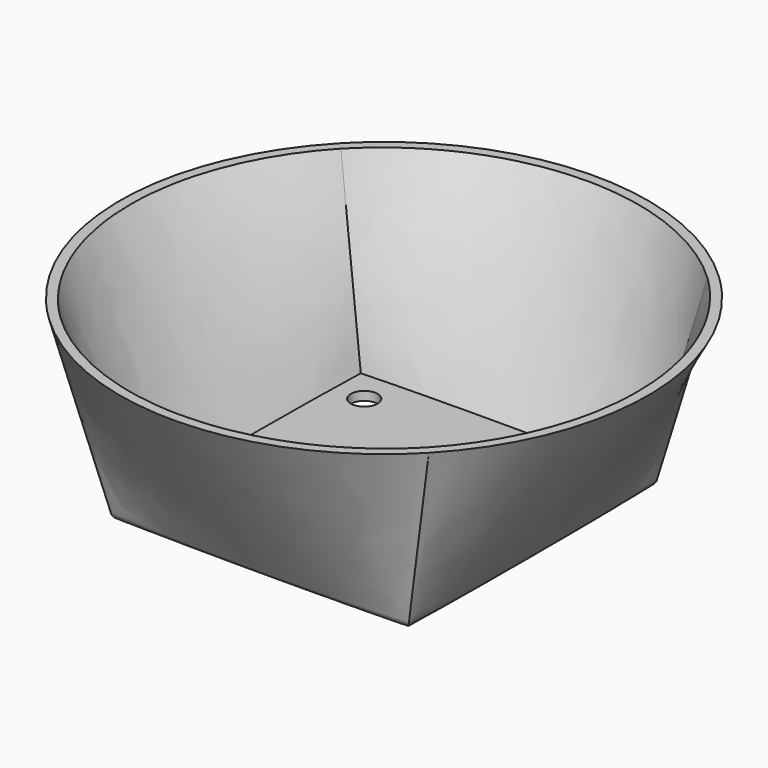
from build123d import *

# Parameters (mm, degrees)
F0_W     = 83.8052779436
F0_H     = 87.6248255372
F4_T     = 2.5
F6_R     = 3.7914698357
F7_DEPTH = 25
F8_R     = 2


# Not quite as in the source:
# - the arcs of a loft's sections are written as splines that run evenly, so that the points pair up as in the source's solid
# - a shell that OpenCascade refuses in one call is made with other operations: the cavity is built on its own and cut out


with BuildPart() as f3:
    # F0 (on Top) → F3 section 0
    with BuildSketch(Plane.XY):
        Rectangle(F0_W, F0_H)
    # F2 (on offset) → F3 section 1
    with BuildSketch(Plane.XY.offset(51.3)):
        with BuildLine():
            add(Edge.make_bspline(
                [(51.8385416369, 54.201158668), (48.2910840976, 57.5939832843), (44.4095584812, 60.6373385743), (36.1271557125, 65.9084541921), (31.7264833589, 68.1360841812), (22.5748809938, 71.6901001672), (17.8241772736, 73.0163982842), (8.1550662585, 74.7167357972), (3.2368980515, 75.0907331491), (-6.5781430996, 74.8720491721), (-11.4747733474, 74.2793732506), (-21.0585581074, 72.1500716861), (-25.7454756417, 70.6134986943), (-34.729704537, 66.6554074074), (-39.0267937453, 64.2339869838), (-47.0662078979, 58.5992132028), (-50.8083340518, 55.3859991763), (-54.201158668, 51.8385416369)],
                knots=[0, 0, 0, 0, 0.125, 0.125, 0.25, 0.25, 0.375, 0.375, 0.5, 0.5, 0.625, 0.625, 0.75, 0.75, 0.875, 0.875, 1, 1, 1, 1], degree=3))
            add(Edge.make_bspline(
                [(-54.201158668, 51.8385416369), (-57.5939832843, 48.2910840976), (-60.6373385743, 44.4095584812), (-65.9084541921, 36.1271557125), (-68.1360841812, 31.7264833589), (-71.6901001672, 22.5748809938), (-73.0163982842, 17.8241772736), (-74.7167357972, 8.1550662585), (-75.0907331491, 3.2368980515), (-74.8720491721, -6.5781430996), (-74.2793732506, -11.4747733474), (-72.1500716861, -21.0585581074), (-70.6134986943, -25.7454756417), (-66.6554074074, -34.729704537), (-64.2339869838, -39.0267937453), (-58.5992132028, -47.0662078979), (-55.3859991763, -50.8083340518), (-51.8385416369, -54.201158668)],
                knots=[0, 0, 0, 0, 0.125, 0.125, 0.25, 0.25, 0.375, 0.375, 0.5, 0.5, 0.625, 0.625, 0.75, 0.75, 0.875, 0.875, 1, 1, 1, 1], degree=3))
            add(Edge.make_bspline(
                [(-51.8385416369, -54.201158668), (-48.2910840976, -57.5939832843), (-44.4095584812, -60.6373385743), (-36.1271557125, -65.9084541921), (-31.7264833589, -68.1360841812), (-22.5748809938, -71.6901001672), (-17.8241772736, -73.0163982842), (-8.1550662585, -74.7167357972), (-3.2368980515, -75.0907331491), (6.5781430996, -74.8720491721), (11.4747733474, -74.2793732506), (21.0585581074, -72.1500716861), (25.7454756417, -70.6134986943), (34.729704537, -66.6554074074), (39.0267937453, -64.2339869838), (47.0662078979, -58.5992132028), (50.8083340518, -55.3859991763), (54.201158668, -51.8385416369)],
                knots=[0, 0, 0, 0, 0.125, 0.125, 0.25, 0.25, 0.375, 0.375, 0.5, 0.5, 0.625, 0.625, 0.75, 0.75, 0.875, 0.875, 1, 1, 1, 1], degree=3))
            add(Edge.make_bspline(
                [(54.201158668, -51.8385416369), (57.5939832843, -48.2910840976), (60.6373385743, -44.4095584812), (65.9084541921, -36.1271557125), (68.1360841812, -31.7264833589), (71.6901001672, -22.5748809938), (73.0163982842, -17.8241772736), (74.7167357972, -8.1550662585), (75.0907331491, -3.2368980515), (74.8720491721, 6.5781430996), (74.2793732506, 11.4747733474), (72.1500716861, 21.0585581074), (70.6134986943, 25.7454756417), (66.6554074074, 34.729704537), (64.2339869838, 39.0267937453), (58.5992132028, 47.0662078979), (55.3859991763, 50.8083340518), (51.8385416369, 54.201158668)],
                knots=[0, 0, 0, 0, 0.125, 0.125, 0.25, 0.25, 0.375, 0.375, 0.5, 0.5, 0.625, 0.625, 0.75, 0.75, 0.875, 0.875, 1, 1, 1, 1], degree=3))
        make_face()
    loft(ruled=True)

    # F4: shell of thickness 2.5, made by hand


with BuildPart() as f4_core1:
    # F4_t2: copy of F3
    add(f3.part)

    # the walls: a layer under each face that stays
    f4_faces = [f4_core1.faces().sort_by_distance(p)[0] for p in [
        (58.4420150662, 0.835311262, 25.65),
        (-0.835311262, 59.3969019646, 25.65),
        (-58.4420150662, -0.835311262, 25.65),
        (0.835311262, -59.3969019646, 25.65),
        (0, 0, 0),
    ]]
    thicken(f4_faces, amount=-F4_T, mode=Mode.SUBTRACT)


with BuildPart() as f3_1:
    add(f3.part)

    # what is left inside the walls is the cavity
    f4_cavity = [f4_core1.part.solids().sort_by_distance(p)[0] for p in [
        (-16.68133, -17.441606, 51.275),
    ]]
    add(f4_cavity, mode=Mode.SUBTRACT)

    # F6 (on face) → F7 (cut)
    with BuildSketch(Plane.XY.offset(2.5)):
        with Locations((-31.7619591951, 32.6714776456)):
            Circle(F6_R)
    extrude(amount=-F7_DEPTH, mode=Mode.SUBTRACT)

    # F8
    f8_edges = [f3_1.edges().sort_by_distance(p)[0] for p in [
        (-41.902639, 0, 0),
        (0, -43.812413, 0),
        (0, 43.812413, 0),
        (41.902639, 0, 0),
    ]]
    fillet(f8_edges, radius=F8_R)


solid = f3_1.part
